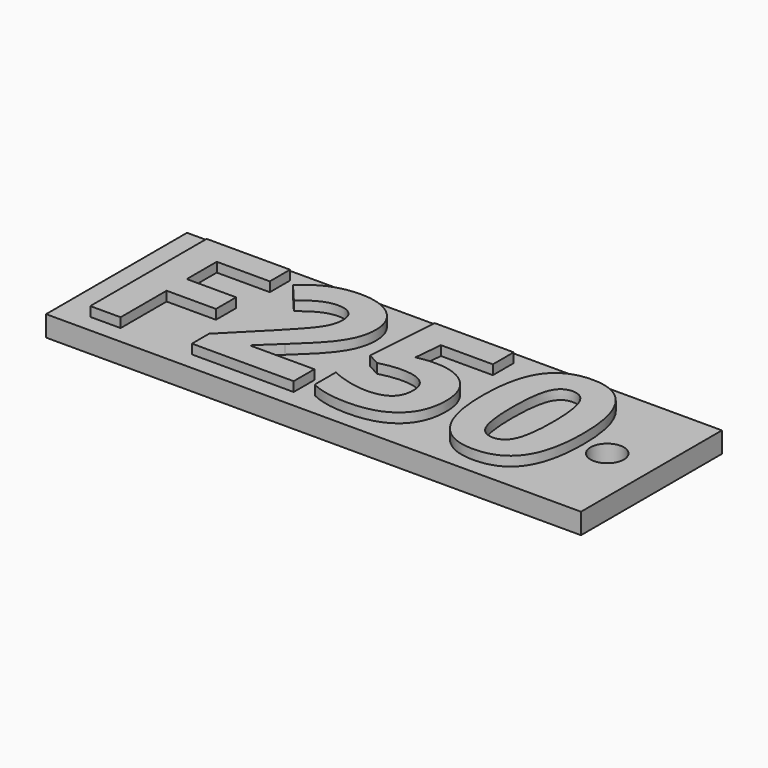
from build123d import *

# Parameters (mm, degrees)
F0_W         = 85.3562876582
F0_H         = 28.1141139567
F1_DEPTH     = 3.302
F2_TEXT_SIZE = 32.5181450333
F3_DEPTH     = 1.524
F4_R         = 2.6564968211
F5_DEPTH     = 13.208


# Not quite as in the source:
# - Text() gives the source's letters only with a copy of the font that has no kerning and outlines rounded to 1/6400 em; it was checked with that copy


with BuildPart() as f1:
    # F0 (on Top) → F1 (new body)
    with BuildSketch(Plane.XY):
        with Locations((-8.1116147339, 14.0570569783)):
            Rectangle(F0_W, F0_H)
    extrude(amount=F1_DEPTH)

    # F2 (on face) → F3 (join)
    with BuildSketch(Plane.XY.offset(3.302)):
        with Locations((-48.9462092519, 2.8575002216)):
            Text('F250', F2_TEXT_SIZE, font='Open Sans', font_style=FontStyle.BOLD, text_align=(TextAlign.LEFT, TextAlign.BOTTOM))
    extrude(amount=F3_DEPTH)

    # F4 (on face) → F5 (cut)
    with BuildSketch(Plane.XY.offset(3.302)):
        with Locations((27.2915810347, 14.329935424)):
            Circle(F4_R)
    extrude(amount=-F5_DEPTH, mode=Mode.SUBTRACT)


solid = f1.part
